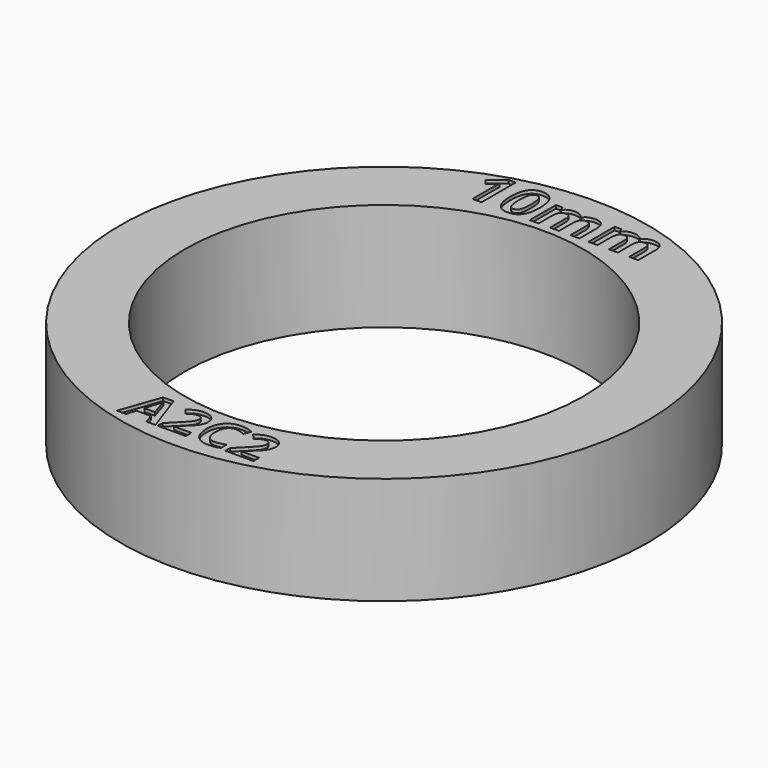
from build123d import *

# Parameters (mm, degrees)
F0_R           = 24.5
F0_R_2         = 18.5
F0_TEXT_SIZE   = 5.1974965673
F0_TEXT_SIZE_2 = 5.5555555556
F1_DEPTH       = 10
F2_DEPTH       = 0.3


# Not quite as in the source:
# - Text() gives the source's letters only with a copy of the font that has no kerning and outlines rounded to 1/6400 em; it was checked with that copy


with BuildPart() as f1:
    # F0 (on Top) → F1 (new body)
    with BuildSketch(Plane.XY):
        Circle(F0_R)
        Polygon((-2.9154707307, -22.8730905801), (-3.7633123583, -22.8730905801), (-4.0321203839, -21.9895161637), (-5.3850937091, -21.9895161637), (-5.6539017347, -22.8730905801), (-6.5017433622, -22.8730905801), (-5.1918118055, -19.1471352284), (-4.2302749405, -19.1471352284), align=None, mode=Mode.SUBTRACT)
        with BuildLine():
            Line((-0.1136952374, -22.2128460943), (-0.1136952374, -22.8730905801))
            Line((-0.1136952374, -22.8730905801), (-2.707570868, -22.8730905801))
            Line((-2.707570868, -22.8730905801), (-2.707570868, -22.3273534405))
            Line((-2.707570868, -22.3273534405), (-1.7760820301, -21.3861192965))
            add(Edge.make_bspline(
                [(-1.7760820301, -21.3861192965), (-1.3619065224, -20.9621984828), (-1.2352175436, -20.7985585518)],
                knots=[0, 0, 0, 1, 1, 1], degree=2))
            add(Edge.make_bspline(
                [(-1.2352175436, -20.7985585518), (-1.1085285648, -20.6349186208), (-1.0524930549, -20.4952359005)],
                knots=[0, 0, 0, 1, 1, 1], degree=2))
            add(Edge.make_bspline(
                [(-1.0524930549, -20.4952359005), (-0.996457545, -20.3555531803), (-0.996457545, -20.206125154)],
                knots=[0, 0, 0, 1, 1, 1], degree=2))
            add(Edge.make_bspline(
                [(-0.996457545, -20.206125154), (-0.996457545, -19.9827952234), (-1.1198980885, -19.8735665846)],
                knots=[0, 0, 0, 1, 1, 1], degree=2))
            add(Edge.make_bspline(
                [(-1.1198980885, -19.8735665846), (-1.243338632, -19.7643379458), (-1.4488021681, -19.7643379458)],
                knots=[0, 0, 0, 1, 1, 1], degree=2))
            add(Edge.make_bspline(
                [(-1.4488021681, -19.7643379458), (-1.6640110104, -19.7643379458), (-1.86703822, -19.8634152241)],
                knots=[0, 0, 0, 1, 1, 1], degree=2))
            add(Edge.make_bspline(
                [(-1.86703822, -19.8634152241), (-2.0700654297, -19.9624925024), (-2.2909590338, -20.1452169911)],
                knots=[0, 0, 0, 1, 1, 1], degree=2))
            Line((-2.2909590338, -20.1452169911), (-2.7173161741, -19.6400852935))
            add(Edge.make_bspline(
                [(-2.7173161741, -19.6400852935), (-2.4436354955, -19.4061979479), (-2.2633473333, -19.3099630505)],
                knots=[0, 0, 0, 1, 1, 1], degree=2))
            add(Edge.make_bspline(
                [(-2.2633473333, -19.3099630505), (-2.0830591711, -19.2137281532), (-1.869880601, -19.1617531875)],
                knots=[0, 0, 0, 1, 1, 1], degree=2))
            add(Edge.make_bspline(
                [(-1.869880601, -19.1617531875), (-1.6567020308, -19.1097782218), (-1.3927666583, -19.1097782218)],
                knots=[0, 0, 0, 1, 1, 1], degree=2))
            add(Edge.make_bspline(
                [(-1.3927666583, -19.1097782218), (-1.0451840753, -19.1097782218), (-0.7788123763, -19.2364672006)],
                knots=[0, 0, 0, 1, 1, 1], degree=2))
            add(Edge.make_bspline(
                [(-0.7788123763, -19.2364672006), (-0.5124406772, -19.3631561795), (-0.365042923, -19.5917648176)],
                knots=[0, 0, 0, 1, 1, 1], degree=2))
            add(Edge.make_bspline(
                [(-0.365042923, -19.5917648176), (-0.2176451688, -19.8203734556), (-0.2176451688, -20.1143568552)],
                knots=[0, 0, 0, 1, 1, 1], degree=2))
            add(Edge.make_bspline(
                [(-0.2176451688, -20.1143568552), (-0.2176451688, -20.3709832482), (-0.3077892498, -20.5955313421)],
                knots=[0, 0, 0, 1, 1, 1], degree=2))
            add(Edge.make_bspline(
                [(-0.3077892498, -20.5955313421), (-0.3979333309, -20.820079436), (-0.5871546903, -21.0559970536)],
                knots=[0, 0, 0, 1, 1, 1], degree=2))
            add(Edge.make_bspline(
                [(-0.5871546903, -21.0559970536), (-0.7763760497, -21.2919146713), (-1.253083938, -21.7288292265)],
                knots=[0, 0, 0, 1, 1, 1], degree=2))
            Line((-1.253083938, -21.7288292265), (-1.7306039352, -22.1779254142))
            Line((-1.7306039352, -22.1779254142), (-1.7306039352, -22.2128460943))
            Line((-1.7306039352, -22.2128460943), (-0.1136952374, -22.2128460943))
        make_face(mode=Mode.SUBTRACT)
        Circle(F0_R_2, mode=Mode.SUBTRACT)
        with BuildLine():
            add(Edge.make_bspline(
                [(2.5077920937, -19.8378337957), (2.2974559045, -19.7643379458), (2.0944286949, -19.7643379458)],
                knots=[0, 0, 0, 1, 1, 1], degree=2))
            add(Edge.make_bspline(
                [(2.0944286949, -19.7643379458), (1.6502051601, -19.7643379458), (1.4065725085, -20.0981146785)],
                knots=[0, 0, 0, 1, 1, 1], degree=2))
            add(Edge.make_bspline(
                [(1.4065725085, -20.0981146785), (1.1629398569, -20.4318914111), (1.1629398569, -21.0279792987)],
                knots=[0, 0, 0, 1, 1, 1], degree=2))
            add(Edge.make_bspline(
                [(1.1629398569, -21.0279792987), (1.1629398569, -22.2688816042), (2.0944286949, -22.2688816042)],
                knots=[0, 0, 0, 1, 1, 1], degree=2))
            add(Edge.make_bspline(
                [(2.0944286949, -22.2688816042), (2.4850530463, -22.2688816042), (3.0405354919, -22.0739754829)],
                knots=[0, 0, 0, 1, 1, 1], degree=2))
            Line((3.0405354919, -22.0739754829), (3.0405354919, -22.7334078599))
            add(Edge.make_bspline(
                [(3.0405354919, -22.7334078599), (2.5841303246, -22.9242534369), (2.0205267906, -22.9242534369)],
                knots=[0, 0, 0, 1, 1, 1], degree=2))
            add(Edge.make_bspline(
                [(2.0205267906, -22.9242534369), (1.2108542784, -22.9242534369), (0.7820608116, -22.4329275896)],
                knots=[0, 0, 0, 1, 1, 1], degree=2))
            add(Edge.make_bspline(
                [(0.7820608116, -22.4329275896), (0.3532673448, -21.9416017422), (0.3532673448, -21.0231066457)],
                knots=[0, 0, 0, 1, 1, 1], degree=2))
            add(Edge.make_bspline(
                [(0.3532673448, -21.0231066457), (0.3532673448, -20.4440730437), (0.5640095884, -20.0087827062)],
                knots=[0, 0, 0, 1, 1, 1], degree=2))
            add(Edge.make_bspline(
                [(0.5640095884, -20.0087827062), (0.7747518321, -19.5734923687), (1.1694367277, -19.3416352953)],
                knots=[0, 0, 0, 1, 1, 1], degree=2))
            add(Edge.make_bspline(
                [(1.1694367277, -19.3416352953), (1.5641216232, -19.1097782218), (2.0944286949, -19.1097782218)],
                knots=[0, 0, 0, 1, 1, 1], degree=2))
            add(Edge.make_bspline(
                [(2.0944286949, -19.1097782218), (2.6344810726, -19.1097782218), (3.1802182121, -19.370465159)],
                knots=[0, 0, 0, 1, 1, 1], degree=2))
            Line((3.1802182121, -19.370465159), (2.9268402545, -20.0104069239))
            add(Edge.make_bspline(
                [(2.9268402545, -20.0104069239), (2.7181282829, -19.9113296456), (2.5077920937, -19.8378337957)],
                knots=[0, 0, 0, 1, 1, 1], degree=2))
        make_face(mode=Mode.SUBTRACT)
        with BuildLine():
            Line((6.1647181942, -22.2128460943), (6.1647181942, -22.8730905801))
            Line((6.1647181942, -22.8730905801), (3.5708425635, -22.8730905801))
            Line((3.5708425635, -22.8730905801), (3.5708425635, -22.3273534405))
            Line((3.5708425635, -22.3273534405), (4.5023314015, -21.3861192965))
            add(Edge.make_bspline(
                [(4.5023314015, -21.3861192965), (4.9165069092, -20.9621984828), (5.043195888, -20.7985585518)],
                knots=[0, 0, 0, 1, 1, 1], degree=2))
            add(Edge.make_bspline(
                [(5.043195888, -20.7985585518), (5.1698848668, -20.6349186208), (5.2259203767, -20.4952359005)],
                knots=[0, 0, 0, 1, 1, 1], degree=2))
            add(Edge.make_bspline(
                [(5.2259203767, -20.4952359005), (5.2819558866, -20.3555531803), (5.2819558866, -20.206125154)],
                knots=[0, 0, 0, 1, 1, 1], degree=2))
            add(Edge.make_bspline(
                [(5.2819558866, -20.206125154), (5.2819558866, -19.9827952234), (5.1585153431, -19.8735665846)],
                knots=[0, 0, 0, 1, 1, 1], degree=2))
            add(Edge.make_bspline(
                [(5.1585153431, -19.8735665846), (5.0350747996, -19.7643379458), (4.8296112634, -19.7643379458)],
                knots=[0, 0, 0, 1, 1, 1], degree=2))
            add(Edge.make_bspline(
                [(4.8296112634, -19.7643379458), (4.6144024212, -19.7643379458), (4.4113752115, -19.8634152241)],
                knots=[0, 0, 0, 1, 1, 1], degree=2))
            add(Edge.make_bspline(
                [(4.4113752115, -19.8634152241), (4.2083480019, -19.9624925024), (3.9874543978, -20.1452169911)],
                knots=[0, 0, 0, 1, 1, 1], degree=2))
            Line((3.9874543978, -20.1452169911), (3.5610972575, -19.6400852935))
            add(Edge.make_bspline(
                [(3.5610972575, -19.6400852935), (3.8347779361, -19.4061979479), (4.0150660983, -19.3099630505)],
                knots=[0, 0, 0, 1, 1, 1], degree=2))
            add(Edge.make_bspline(
                [(4.0150660983, -19.3099630505), (4.1953542604, -19.2137281532), (4.4085328306, -19.1617531875)],
                knots=[0, 0, 0, 1, 1, 1], degree=2))
            add(Edge.make_bspline(
                [(4.4085328306, -19.1617531875), (4.6217114007, -19.1097782218), (4.8856467733, -19.1097782218)],
                knots=[0, 0, 0, 1, 1, 1], degree=2))
            add(Edge.make_bspline(
                [(4.8856467733, -19.1097782218), (5.2332293562, -19.1097782218), (5.4996010553, -19.2364672006)],
                knots=[0, 0, 0, 1, 1, 1], degree=2))
            add(Edge.make_bspline(
                [(5.4996010553, -19.2364672006), (5.7659727544, -19.3631561795), (5.9133705086, -19.5917648176)],
                knots=[0, 0, 0, 1, 1, 1], degree=2))
            add(Edge.make_bspline(
                [(5.9133705086, -19.5917648176), (6.0607682628, -19.8203734556), (6.0607682628, -20.1143568552)],
                knots=[0, 0, 0, 1, 1, 1], degree=2))
            add(Edge.make_bspline(
                [(6.0607682628, -20.1143568552), (6.0607682628, -20.3709832482), (5.9706241817, -20.5955313421)],
                knots=[0, 0, 0, 1, 1, 1], degree=2))
            add(Edge.make_bspline(
                [(5.9706241817, -20.5955313421), (5.8804801006, -20.820079436), (5.6912587412, -21.0559970536)],
                knots=[0, 0, 0, 1, 1, 1], degree=2))
            add(Edge.make_bspline(
                [(5.6912587412, -21.0559970536), (5.5020373818, -21.2919146713), (5.0253294935, -21.7288292265)],
                knots=[0, 0, 0, 1, 1, 1], degree=2))
            Line((5.0253294935, -21.7288292265), (4.5478094964, -22.1779254142))
            Line((4.5478094964, -22.1779254142), (4.5478094964, -22.2128460943))
            Line((4.5478094964, -22.2128460943), (6.1647181942, -22.2128460943))
        make_face(mode=Mode.SUBTRACT)
        with BuildLine():
            Line((-6.3033854167, 23.1475137876), (-6.3033854167, 19.1813679542))
            Line((-6.3033854167, 19.1813679542), (-7.1419270833, 19.1813679542))
            Line((-7.1419270833, 19.1813679542), (-7.1419270833, 21.4765068431))
            Line((-7.1419270833, 21.4765068431), (-7.1332465278, 21.8532429542))
            Line((-7.1332465278, 21.8532429542), (-7.1202256944, 22.2655693431))
            add(Edge.make_bspline(
                [(-7.1202256944, 22.2655693431), (-7.3285590278, 22.0572360098), (-7.41015625, 21.9921318431)],
                knots=[0, 0, 0, 1, 1, 1], degree=2))
            Line((-7.41015625, 21.9921318431), (-7.8658854167, 21.6258123987))
            Line((-7.8658854167, 21.6258123987), (-8.2703993056, 22.1301526765))
            Line((-8.2703993056, 22.1301526765), (-6.9926215278, 23.1475137876))
            Line((-6.9926215278, 23.1475137876), (-6.3033854167, 23.1475137876))
        make_face(mode=Mode.SUBTRACT)
        with BuildLine():
            add(Edge.make_bspline(
                [(-2.8055555556, 22.6891804542), (-2.4544270833, 22.1683471209), (-2.4544270833, 21.1640068431)],
                knots=[0, 0, 0, 1, 1, 1], degree=2))
            add(Edge.make_bspline(
                [(-2.4544270833, 21.1640068431), (-2.4544270833, 20.1258123987), (-2.7947048611, 19.6262464265)],
                knots=[0, 0, 0, 1, 1, 1], degree=2))
            add(Edge.make_bspline(
                [(-2.7947048611, 19.6262464265), (-3.1349826389, 19.1266804542), (-3.8433159722, 19.1266804542)],
                knots=[0, 0, 0, 1, 1, 1], degree=2))
            add(Edge.make_bspline(
                [(-3.8433159722, 19.1266804542), (-4.5299479167, 19.1266804542), (-4.8784722222, 19.6423054542)],
                knots=[0, 0, 0, 1, 1, 1], degree=2))
            add(Edge.make_bspline(
                [(-4.8784722222, 19.6423054542), (-5.2269965278, 20.1579304542), (-5.2269965278, 21.1640068431)],
                knots=[0, 0, 0, 1, 1, 1], degree=2))
            add(Edge.make_bspline(
                [(-5.2269965278, 21.1640068431), (-5.2269965278, 22.2143540654), (-4.8875868056, 22.7121839265)],
                knots=[0, 0, 0, 1, 1, 1], degree=2))
            add(Edge.make_bspline(
                [(-4.8875868056, 22.7121839265), (-4.5481770833, 23.2100137876), (-3.8433159722, 23.2100137876)],
                knots=[0, 0, 0, 1, 1, 1], degree=2))
            add(Edge.make_bspline(
                [(-3.8433159722, 23.2100137876), (-3.1566840278, 23.2100137876), (-2.8055555556, 22.6891804542)],
                knots=[0, 0, 0, 1, 1, 1], degree=2))
        make_face(mode=Mode.SUBTRACT)
        with BuildLine():
            Line((0.8927951389, 20.7030693431), (0.8927951389, 19.1813679542))
            Line((0.8927951389, 19.1813679542), (0.0655381944, 19.1813679542))
            Line((0.0655381944, 19.1813679542), (0.0655381944, 20.9530693431))
            add(Edge.make_bspline(
                [(0.0655381944, 20.9530693431), (0.0655381944, 21.2811943431), (-0.0442708333, 21.4452568431)],
                knots=[0, 0, 0, 1, 1, 1], degree=2))
            add(Edge.make_bspline(
                [(-0.0442708333, 21.4452568431), (-0.1540798611, 21.6093193431), (-0.3901909722, 21.6093193431)],
                knots=[0, 0, 0, 1, 1, 1], degree=2))
            add(Edge.make_bspline(
                [(-0.3901909722, 21.6093193431), (-0.7078993056, 21.6093193431), (-0.8515625, 21.3758123987)],
                knots=[0, 0, 0, 1, 1, 1], degree=2))
            add(Edge.make_bspline(
                [(-0.8515625, 21.3758123987), (-0.9952256944, 21.1423054542), (-0.9952256944, 20.6084512876)],
                knots=[0, 0, 0, 1, 1, 1], degree=2))
            Line((-0.9952256944, 20.6084512876), (-0.9952256944, 19.1813679542))
            Line((-0.9952256944, 19.1813679542), (-1.8224826389, 19.1813679542))
            Line((-1.8224826389, 19.1813679542), (-1.8224826389, 22.2143540654))
            Line((-1.8224826389, 22.2143540654), (-1.1905381944, 22.2143540654))
            Line((-1.1905381944, 22.2143540654), (-1.0794270833, 21.826333232))
            Line((-1.0794270833, 21.826333232), (-1.0334201389, 21.826333232))
            add(Edge.make_bspline(
                [(-1.0334201389, 21.826333232), (-0.9110243056, 22.0355346209), (-0.6805555556, 22.1531561487)],
                knots=[0, 0, 0, 1, 1, 1], degree=2))
            add(Edge.make_bspline(
                [(-0.6805555556, 22.1531561487), (-0.4500868056, 22.2707776765), (-0.1514756944, 22.2707776765)],
                knots=[0, 0, 0, 1, 1, 1], degree=2))
            add(Edge.make_bspline(
                [(-0.1514756944, 22.2707776765), (0.5290798611, 22.2707776765), (0.7712673611, 21.826333232)],
                knots=[0, 0, 0, 1, 1, 1], degree=2))
            Line((0.7712673611, 21.826333232), (0.8441840278, 21.826333232))
            add(Edge.make_bspline(
                [(0.8441840278, 21.826333232), (0.9665798611, 22.0381387876), (1.2035590278, 22.154458232)],
                knots=[0, 0, 0, 1, 1, 1], degree=2))
            add(Edge.make_bspline(
                [(1.2035590278, 22.154458232), (1.4405381944, 22.2707776765), (1.7391493056, 22.2707776765)],
                knots=[0, 0, 0, 1, 1, 1], degree=2))
            add(Edge.make_bspline(
                [(1.7391493056, 22.2707776765), (2.2547743056, 22.2707776765), (2.5190972222, 22.0064547598)],
                knots=[0, 0, 0, 1, 1, 1], degree=2))
            add(Edge.make_bspline(
                [(2.5190972222, 22.0064547598), (2.7834201389, 21.7421318431), (2.7834201389, 21.1587985098)],
                knots=[0, 0, 0, 1, 1, 1], degree=2))
            Line((2.7834201389, 21.1587985098), (2.7834201389, 19.1813679542))
            Line((2.7834201389, 19.1813679542), (1.9535590278, 19.1813679542))
            Line((1.9535590278, 19.1813679542), (1.9535590278, 20.9530693431))
            add(Edge.make_bspline(
                [(1.9535590278, 20.9530693431), (1.9535590278, 21.2811943431), (1.84375, 21.4452568431)],
                knots=[0, 0, 0, 1, 1, 1], degree=2))
            add(Edge.make_bspline(
                [(1.84375, 21.4452568431), (1.7339409722, 21.6093193431), (1.4978298611, 21.6093193431)],
                knots=[0, 0, 0, 1, 1, 1], degree=2))
            add(Edge.make_bspline(
                [(1.4978298611, 21.6093193431), (1.1940104167, 21.6093193431), (1.0434027778, 21.3923054542)],
                knots=[0, 0, 0, 1, 1, 1], degree=2))
            add(Edge.make_bspline(
                [(1.0434027778, 21.3923054542), (0.8927951389, 21.1752915654), (0.8927951389, 20.7030693431)],
                knots=[0, 0, 0, 1, 1, 1], degree=2))
        make_face(mode=Mode.SUBTRACT)
        with BuildLine():
            Line((6.34765625, 20.7030693431), (6.34765625, 19.1813679542))
            Line((6.34765625, 19.1813679542), (5.5203993056, 19.1813679542))
            Line((5.5203993056, 19.1813679542), (5.5203993056, 20.9530693431))
            add(Edge.make_bspline(
                [(5.5203993056, 20.9530693431), (5.5203993056, 21.2811943431), (5.4105902778, 21.4452568431)],
                knots=[0, 0, 0, 1, 1, 1], degree=2))
            add(Edge.make_bspline(
                [(5.4105902778, 21.4452568431), (5.30078125, 21.6093193431), (5.0646701389, 21.6093193431)],
                knots=[0, 0, 0, 1, 1, 1], degree=2))
            add(Edge.make_bspline(
                [(5.0646701389, 21.6093193431), (4.7469618056, 21.6093193431), (4.6032986111, 21.3758123987)],
                knots=[0, 0, 0, 1, 1, 1], degree=2))
            add(Edge.make_bspline(
                [(4.6032986111, 21.3758123987), (4.4596354167, 21.1423054542), (4.4596354167, 20.6084512876)],
                knots=[0, 0, 0, 1, 1, 1], degree=2))
            Line((4.4596354167, 20.6084512876), (4.4596354167, 19.1813679542))
            Line((4.4596354167, 19.1813679542), (3.6323784722, 19.1813679542))
            Line((3.6323784722, 19.1813679542), (3.6323784722, 22.2143540654))
            Line((3.6323784722, 22.2143540654), (4.2643229167, 22.2143540654))
            Line((4.2643229167, 22.2143540654), (4.3754340278, 21.826333232))
            Line((4.3754340278, 21.826333232), (4.4214409722, 21.826333232))
            add(Edge.make_bspline(
                [(4.4214409722, 21.826333232), (4.5438368056, 22.0355346209), (4.7743055556, 22.1531561487)],
                knots=[0, 0, 0, 1, 1, 1], degree=2))
            add(Edge.make_bspline(
                [(4.7743055556, 22.1531561487), (5.0047743056, 22.2707776765), (5.3033854167, 22.2707776765)],
                knots=[0, 0, 0, 1, 1, 1], degree=2))
            add(Edge.make_bspline(
                [(5.3033854167, 22.2707776765), (5.9839409722, 22.2707776765), (6.2261284722, 21.826333232)],
                knots=[0, 0, 0, 1, 1, 1], degree=2))
            Line((6.2261284722, 21.826333232), (6.2990451389, 21.826333232))
            add(Edge.make_bspline(
                [(6.2990451389, 21.826333232), (6.4214409722, 22.0381387876), (6.6584201389, 22.154458232)],
                knots=[0, 0, 0, 1, 1, 1], degree=2))
            add(Edge.make_bspline(
                [(6.6584201389, 22.154458232), (6.8953993056, 22.2707776765), (7.1940104167, 22.2707776765)],
                knots=[0, 0, 0, 1, 1, 1], degree=2))
            add(Edge.make_bspline(
                [(7.1940104167, 22.2707776765), (7.7096354167, 22.2707776765), (7.9739583333, 22.0064547598)],
                knots=[0, 0, 0, 1, 1, 1], degree=2))
            add(Edge.make_bspline(
                [(7.9739583333, 22.0064547598), (8.23828125, 21.7421318431), (8.23828125, 21.1587985098)],
                knots=[0, 0, 0, 1, 1, 1], degree=2))
            Line((8.23828125, 21.1587985098), (8.23828125, 19.1813679542))
            Line((8.23828125, 19.1813679542), (7.4084201389, 19.1813679542))
            Line((7.4084201389, 19.1813679542), (7.4084201389, 20.9530693431))
            add(Edge.make_bspline(
                [(7.4084201389, 20.9530693431), (7.4084201389, 21.2811943431), (7.2986111111, 21.4452568431)],
                knots=[0, 0, 0, 1, 1, 1], degree=2))
            add(Edge.make_bspline(
                [(7.2986111111, 21.4452568431), (7.1888020833, 21.6093193431), (6.9526909722, 21.6093193431)],
                knots=[0, 0, 0, 1, 1, 1], degree=2))
            add(Edge.make_bspline(
                [(6.9526909722, 21.6093193431), (6.6488715278, 21.6093193431), (6.4982638889, 21.3923054542)],
                knots=[0, 0, 0, 1, 1, 1], degree=2))
            add(Edge.make_bspline(
                [(6.4982638889, 21.3923054542), (6.34765625, 21.1752915654), (6.34765625, 20.7030693431)],
                knots=[0, 0, 0, 1, 1, 1], degree=2))
        make_face(mode=Mode.SUBTRACT)
        with BuildLine():
            Line((-5.1869391524, -21.3300837867), (-4.2205296344, -21.3300837867))
            add(Edge.make_bspline(
                [(-4.2205296344, -21.3300837867), (-4.5932875914, -20.1297869232), (-4.640389904, -19.9722378085)],
                knots=[0, 0, 0, 1, 1, 1], degree=2))
            add(Edge.make_bspline(
                [(-4.640389904, -19.9722378085), (-4.6874922167, -19.8146886938), (-4.7077949376, -19.7237325038)],
                knots=[0, 0, 0, 1, 1, 1], degree=2))
            add(Edge.make_bspline(
                [(-4.7077949376, -19.7237325038), (-4.791442148, -20.0485760393), (-5.1869391524, -21.3300837867)],
                knots=[0, 0, 0, 1, 1, 1], degree=2))
        make_face()
        with Locations((-6.5017433622, -22.8730905801)):
            Text('A2C2', F0_TEXT_SIZE, font='Open Sans', font_style=FontStyle.BOLD, text_align=(TextAlign.LEFT, TextAlign.BOTTOM))
        with BuildLine():
            add(Edge.make_bspline(
                [(-4.2664930556, 22.2126179542), (-4.3936631944, 21.8940415654), (-4.3936631944, 21.1640068431)],
                knots=[0, 0, 0, 1, 1, 1], degree=2))
            add(Edge.make_bspline(
                [(-4.3936631944, 21.1640068431), (-4.3936631944, 20.4348401765), (-4.2677951389, 20.1188679542)],
                knots=[0, 0, 0, 1, 1, 1], degree=2))
            add(Edge.make_bspline(
                [(-4.2677951389, 20.1188679542), (-4.1419270833, 19.802895732), (-3.8433159722, 19.802895732)],
                knots=[0, 0, 0, 1, 1, 1], degree=2))
            add(Edge.make_bspline(
                [(-3.8433159722, 19.802895732), (-3.5499131944, 19.802895732), (-3.4197048611, 20.1227742042)],
                knots=[0, 0, 0, 1, 1, 1], degree=2))
            add(Edge.make_bspline(
                [(-3.4197048611, 20.1227742042), (-3.2894965278, 20.4426526765), (-3.2894965278, 21.1640068431)],
                knots=[0, 0, 0, 1, 1, 1], degree=2))
            add(Edge.make_bspline(
                [(-3.2894965278, 21.1640068431), (-3.2894965278, 21.8940415654), (-3.4214409722, 22.2126179542)],
                knots=[0, 0, 0, 1, 1, 1], degree=2))
            add(Edge.make_bspline(
                [(-3.4214409722, 22.2126179542), (-3.5533854167, 22.5311943431), (-3.8433159722, 22.5311943431)],
                knots=[0, 0, 0, 1, 1, 1], degree=2))
            add(Edge.make_bspline(
                [(-3.8433159722, 22.5311943431), (-4.1393229167, 22.5311943431), (-4.2664930556, 22.2126179542)],
                knots=[0, 0, 0, 1, 1, 1], degree=2))
        make_face()
        with Locations((-8.5985243056, 19.1813679542)):
            Text('10mm', F0_TEXT_SIZE_2, font='Open Sans', font_style=FontStyle.BOLD, text_align=(TextAlign.LEFT, TextAlign.BOTTOM))
    extrude(amount=-F1_DEPTH)

    # F0 (on Top) → F2 (cut)
    with BuildSketch(Plane.XY):
        with Locations((-6.5017433622, -22.8730905801)):
            Text('A2C2', F0_TEXT_SIZE, font='Open Sans', font_style=FontStyle.BOLD, text_align=(TextAlign.LEFT, TextAlign.BOTTOM))
        with Locations((-8.5985243056, 19.1813679542)):
            Text('10mm', F0_TEXT_SIZE_2, font='Open Sans', font_style=FontStyle.BOLD, text_align=(TextAlign.LEFT, TextAlign.BOTTOM))
    extrude(amount=-F2_DEPTH, mode=Mode.SUBTRACT)


solid = f1.part
